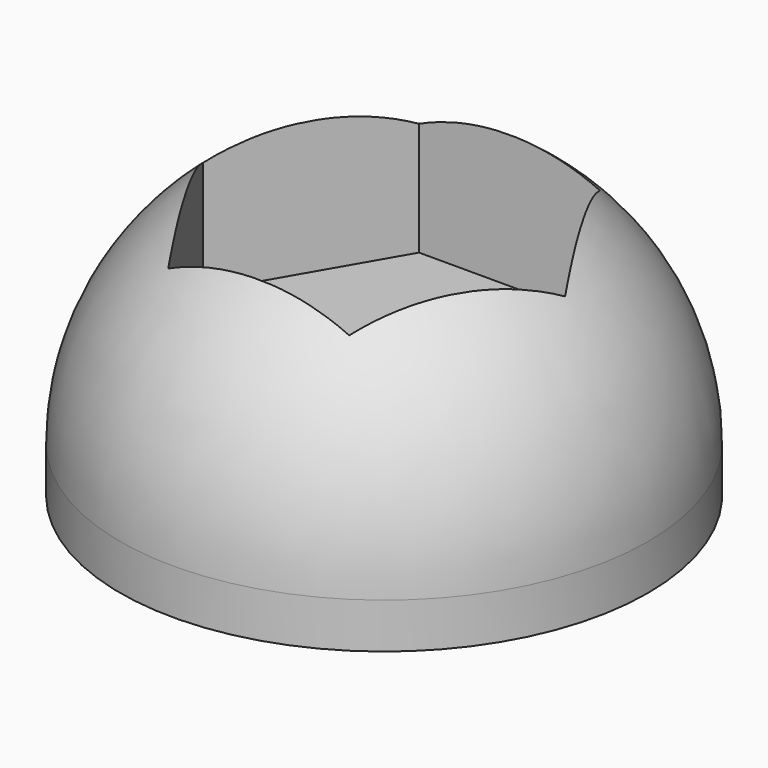
from build123d import *

# Parameters (mm, degrees)
F0_R     = 17.5
F1_DEPTH = 20
F3_DEPTH = 12


# Not quite as in the source:
# - a fillet or chamfer that OpenCascade refuses, or shapes differently, is made with other operations: its cross-section is extruded or revolved along the edge and cut away or added


with BuildPart() as f1:
    # F0 (on Top) → F1 (new body)
    with BuildSketch(Plane.XY):
        Circle(F0_R)
    extrude(amount=F1_DEPTH)

    # F2 (on face) → F3 (cut)
    with BuildSketch(Plane.XY.offset(20)):
        Polygon((6, 10.3923048454), (-6, 10.3923048454), (-12, 0), (-6, -10.3923048454), (6, -10.3923048454), (12, 0), align=None)
    extrude(amount=-F3_DEPTH, mode=Mode.SUBTRACT)

    # F4: fillet of radius 17 on 1 edges, made by hand

    # F4_s1 → F4_t2 (revolve, cut)
    with BuildSketch(Plane.XZ):
        with BuildLine():
            ThreePointArc((17.5, 3), (12.5208152802, 15.0208152802), (0.5, 20))
            Line((0.5, 20), (17.5, 20))
            Line((17.5, 20), (17.5, 3))
        make_face()
    revolve(axis=Axis((0, 0, 20), (0, 0, 1)), mode=Mode.SUBTRACT)


solid = f1.part
